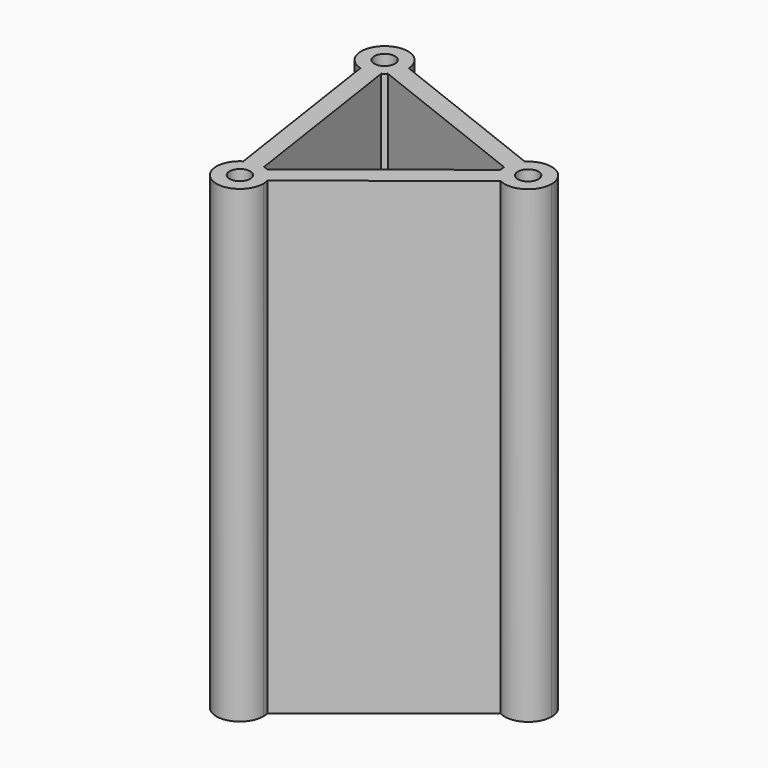
from build123d import *

# Parameters (mm, degrees)
F2_DEPTH = 500
F4_D     = 22
F4_DEPTH = 500
F4_TIP   = 6.6094668093


with BuildPart() as f2:
    # F1 (on Top) → F2 (new body)
    with BuildSketch(Plane.XY):
        with BuildLine():
            ThreePointArc((-163.0534820056, 70.1662666553), (-157.6223484782, 78.2824576852), (-155.7149531136, 87.8601197772))
            ThreePointArc((-155.7149531136, 87.8601197772), (-155.7191665297, 88.3190893279), (-155.7318053575, 88.7779041722))
            ThreePointArc((-155.7318053575, 88.7779041722), (-196.2865938282, 107.4183406948), (-187.2075438541, 63.7179105685))
            ThreePointArc((-187.2075438541, 63.7179105685), (-177.008627135, 63.1363832526), (-167.4285546343, 66.6829713514))
            ThreePointArc((-167.4285546343, 66.6829713514), (-165.1433123991, 68.3018988597), (-163.0534820056, 70.1662666553))
        make_face()
        with BuildLine():
            ThreePointArc((-167.4285546343, 66.6829713514), (-177.008627135, 63.1363832526), (-187.2075438541, 63.7179105685))
            Line((-187.2075438541, 63.7179105685), (-158.4206221982, -128.3106024335))
            ThreePointArc((-158.4206221982, -128.3106024335), (-148.8405496975, -124.7640143347), (-138.6416329785, -125.3455416506))
            Line((-138.6416329785, -125.3455416506), (-167.4285546343, 66.6829713514))
        make_face()
        with BuildLine():
            ThreePointArc((-138.6416329785, -125.3455416506), (-148.8405496975, -124.7640143347), (-158.4206221982, -128.3106024335))
            ThreePointArc((-158.4206221982, -128.3106024335), (-157.2346377204, -171.364221804), (-120.1342237189, -149.4877508594))
            ThreePointArc((-120.1342237189, -149.4877508594), (-120.346610419, -146.2359472222), (-120.9801618704, -143.0393947726))
            ThreePointArc((-120.9801618704, -143.0393947726), (-125.5760028014, -133.9161101448), (-133.437474442, -127.3928180386))
            ThreePointArc((-133.437474442, -127.3928180386), (-135.9821279087, -126.2232039632), (-138.6416329785, -125.3455416506))
        make_face()
        with BuildLine():
            ThreePointArc((30.9279478124, -22.0949328208), (23.0664761717, -15.5716407145), (18.4706352408, -6.4483560868))
            Line((18.4706352408, -6.4483560868), (-133.437474442, -127.3928180386))
            ThreePointArc((-133.437474442, -127.3928180386), (-125.5760028014, -133.9161101448), (-120.9801618704, -143.0393947726))
            Line((-120.9801618704, -143.0393947726), (30.9279478124, -22.0949328208))
        make_face()
        with BuildLine():
            ThreePointArc((67.6246970892, 0), (52.2023591813, 23.0926046355), (24.9632259812, 17.6938531219))
            ThreePointArc((24.9632259812, 17.6938531219), (19.3601501931, 9.1520958101), (17.6415493331, -0.917784395))
            ThreePointArc((17.6415493331, -0.917784395), (17.9009605645, -3.7063259786), (18.4706352408, -6.4483560868))
            ThreePointArc((18.4706352408, -6.4483560868), (23.0664761717, -15.5716407145), (30.9279478124, -22.0949328208))
            ThreePointArc((30.9279478124, -22.0949328208), (55.5200696716, -21.417501394), (67.6246970892, 0))
        make_face()
        with BuildLine():
            ThreePointArc((-155.7318053575, 88.7779041722), (-155.7191665297, 88.3190893279), (-155.7149531136, 87.8601197772))
            ThreePointArc((-155.7149531136, 87.8601197772), (-157.6223484782, 78.2824576852), (-163.0534820056, 70.1662666553))
            Line((-163.0534820056, 70.1662666553), (17.6415493331, -0.917784395))
            ThreePointArc((17.6415493331, -0.917784395), (19.3601501931, 9.1520958101), (24.9632259812, 17.6938531219))
            Line((24.9632259812, 17.6938531219), (-155.7318053575, 88.7779041722))
        make_face()
    extrude(amount=F2_DEPTH)

    # F4
    with Locations(Plane.XY.offset(500)):
        with Locations((-180.7149531136, 87.8601197772), (42.6246970892, 0), (-145.1342237189, -149.4877508594)):
            Hole(F4_D / 2, depth=F4_DEPTH)
            with Locations((0, 0, -(F4_DEPTH + F4_TIP / 2))):  # 118° drill point
                Cone(0, F4_D / 2, F4_TIP, mode=Mode.SUBTRACT)


solid = f2.part
